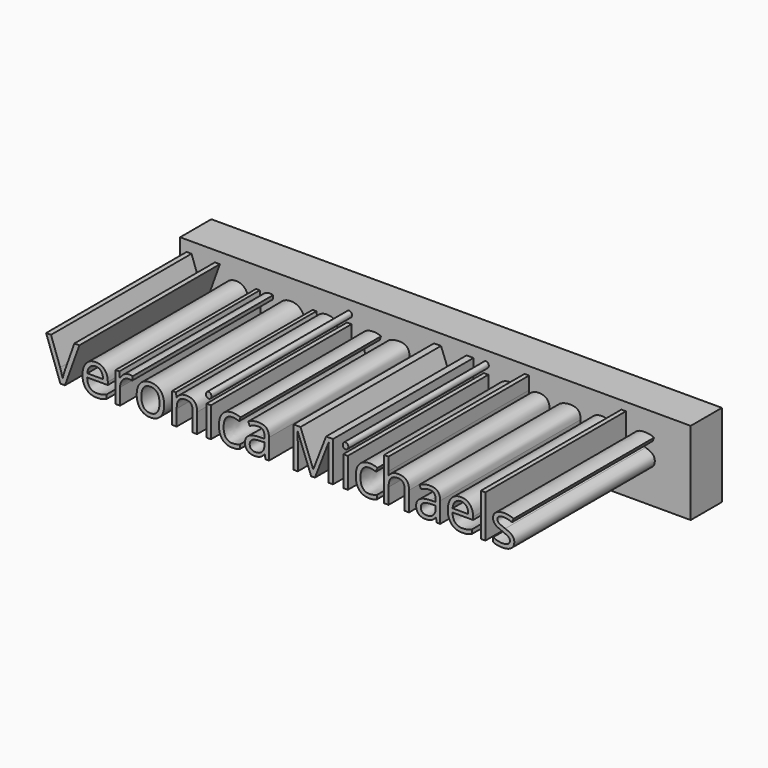
from build123d import *

# Parameters (mm, degrees)
F0_W         = 332.2657123208
F0_H         = 53.9961196482
F1_DEPTH     = 25.4
F2_TEXT_SIZE = 36.3841989181
F3_DEPTH     = 114.3


# Not quite as in the source:
# - Text() gives the source's letters only with a copy of the font that has no kerning and outlines rounded to 1/6400 em; it was checked with that copy


with BuildPart() as f1:
    # F0 (on Front) → F1 (new body)
    with BuildSketch(Plane.XZ):
        with Locations((87.723236531, 26.9980598241)):
            Rectangle(F0_W, F0_H)
    extrude(amount=F1_DEPTH)

    # F2 (on face) → F3 (join)
    with BuildSketch(Plane.XZ.offset(25.4)):
        with Locations((-74.2002725601, 20.9778528661)):
            Text('Veronica Michaels', F2_TEXT_SIZE, font='Open Sans', text_align=(TextAlign.LEFT, TextAlign.BOTTOM))
    extrude(amount=F3_DEPTH)


solid = f1.part
